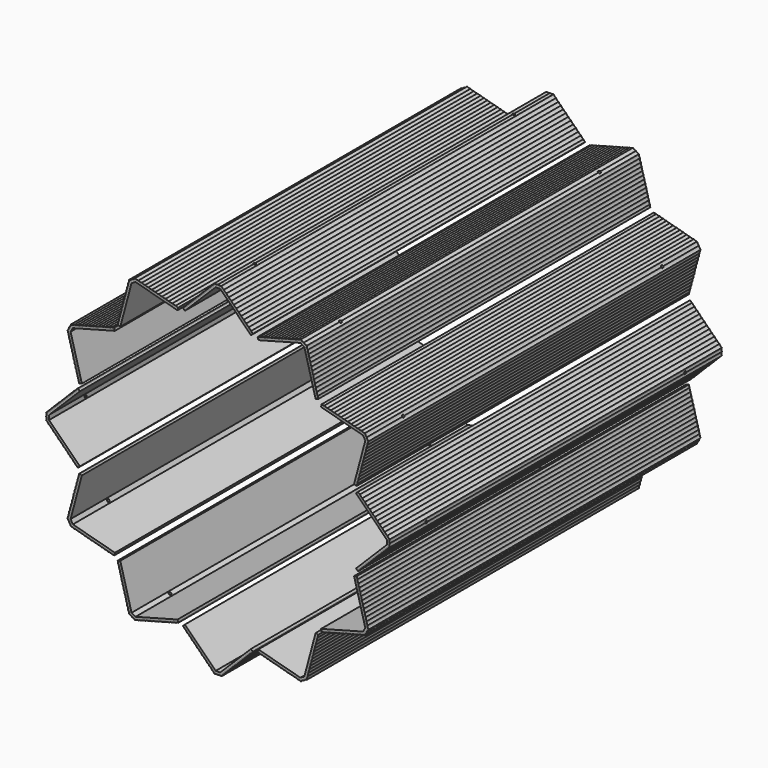
from build123d import *

# Parameters (mm, degrees)
F1_DEPTH = 749.3
F2_DEPTH = 749.3
F3_DEPTH = 749.3
F4_R     = 4.7625
F5_DEPTH = 10.8341
F7_COUNT = 12


with BuildPart() as f1:
    # F0 (on Front) → F1 (new body, symmetric)
    with BuildSketch(Plane.XZ):
        Polygon((8.2127830575, 0), (0, 0), (-8.2127830575, 0), (-119.3411055301, 111.1283224727), (-123.5887666754, 106.8806613274), (-10.701005348, -6.0071), (0, -6.0071), (10.701005348, -6.0071), (123.5887666754, 106.8806613274), (119.3411055301, 111.1283224727), align=None)
        with BuildLine():
            Line((126.3344906062, 104.1349373966), (124.3071871651, 106.1622408377))
            Line((124.3071871651, 106.1622408377), (11.1218463274, -7.0231))
            Line((11.1218463274, -7.0231), (0, -7.0231))
            Line((0, -7.0231), (-11.1218463274, -7.0231))
            Line((-11.1218463274, -7.0231), (-124.3071871651, 106.1622408377))
            Line((-124.3071871651, 106.1622408377), (-126.3344906062, 104.1349373966))
            ThreePointArc((-126.3344906062, 104.1349373966), (-122.9158165988, 100.9260301236), (-120.4630734528, 96.9299734528))
            ThreePointArc((-120.4630734528, 96.9299734528), (-115.136915248, 93.2758755366), (-111.4828173318, 87.9497173318))
            ThreePointArc((-111.4828173318, 87.9497173318), (-106.1566591269, 84.2956194155), (-102.5025612107, 78.9694612107))
            ThreePointArc((-102.5025612107, 78.9694612107), (-97.1764030059, 75.3153632944), (-93.5223050896, 69.9892050896))
            ThreePointArc((-93.5223050896, 69.9892050896), (-88.1961468848, 66.3351071734), (-84.5420489686, 61.0089489686))
            ThreePointArc((-84.5420489686, 61.0089489686), (-79.2158907637, 57.3548510523), (-75.5617928475, 52.0286928475))
            ThreePointArc((-75.5617928475, 52.0286928475), (-70.2356346427, 48.3745949312), (-66.5815367264, 43.0484367264))
            ThreePointArc((-66.5815367264, 43.0484367264), (-61.2553785216, 39.3943388102), (-57.6012806053, 34.0681806053))
            ThreePointArc((-57.6012806053, 34.0681806053), (-52.2751224005, 30.4140826891), (-48.6210244843, 25.0879244843))
            ThreePointArc((-48.6210244843, 25.0879244843), (-43.2948662795, 21.433826568), (-39.6407683632, 16.1076683632))
            ThreePointArc((-39.6407683632, 16.1076683632), (-34.3146101584, 12.453570447), (-30.6605122421, 7.1274122421))
            ThreePointArc((-30.6605122421, 7.1274122421), (-25.3343540373, 3.4733143259), (-21.6802561211, -1.8528438789))
            ThreePointArc((-21.6802561211, -1.8528438789), (-16.3540979162, -5.5069417952), (-12.7, -10.8331))
            ThreePointArc((-12.7, -10.8331), (-6.35, -9.6507748314), (0, -10.8331))
            ThreePointArc((0, -10.8331), (6.35, -9.6507748314), (12.7, -10.8331))
            ThreePointArc((12.7, -10.8331), (16.3540979162, -5.5069417952), (21.6802561211, -1.8528438789))
            ThreePointArc((21.6802561211, -1.8528438789), (25.3343540373, 3.4733143259), (30.6605122421, 7.1274122421))
            ThreePointArc((30.6605122421, 7.1274122421), (34.3146101584, 12.453570447), (39.6407683632, 16.1076683632))
            ThreePointArc((39.6407683632, 16.1076683632), (43.2948662795, 21.433826568), (48.6210244843, 25.0879244843))
            ThreePointArc((48.6210244843, 25.0879244843), (52.2751224005, 30.4140826891), (57.6012806053, 34.0681806053))
            ThreePointArc((57.6012806053, 34.0681806053), (61.2553785216, 39.3943388102), (66.5815367264, 43.0484367264))
            ThreePointArc((66.5815367264, 43.0484367264), (70.2356346427, 48.3745949312), (75.5617928475, 52.0286928475))
            ThreePointArc((75.5617928475, 52.0286928475), (79.2158907637, 57.3548510523), (84.5420489686, 61.0089489686))
            ThreePointArc((84.5420489686, 61.0089489686), (88.1961468848, 66.3351071734), (93.5223050896, 69.9892050896))
            ThreePointArc((93.5223050896, 69.9892050896), (97.1764030059, 75.3153632944), (102.5025612107, 78.9694612107))
            ThreePointArc((102.5025612107, 78.9694612107), (106.1566591269, 84.2956194155), (111.4828173318, 87.9497173318))
            ThreePointArc((111.4828173318, 87.9497173318), (115.136915248, 93.2758755366), (120.4630734528, 96.9299734528))
            ThreePointArc((120.4630734528, 96.9299734528), (122.9158165988, 100.9260301236), (126.3344906062, 104.1349373966))
        make_face()
        Polygon((124.3071871651, 106.1622408377), (123.5887666754, 106.8806613274), (10.701005348, -6.0071), (0, -6.0071), (-10.701005348, -6.0071), (-123.5887666754, 106.8806613274), (-124.3071871651, 106.1622408377), (-11.1218463274, -7.0231), (0, -7.0231), (11.1218463274, -7.0231), align=None)
    extrude(amount=F1_DEPTH, both=True)


with BuildPart() as f2:
    # F0 (on Front) → F2 (new body, symmetric)
    with BuildSketch(Plane.XZ):
        Polygon((124.3071871651, 106.1622408377), (123.5887666754, 106.8806613274), (10.701005348, -6.0071), (0, -6.0071), (-10.701005348, -6.0071), (-123.5887666754, 106.8806613274), (-124.3071871651, 106.1622408377), (-11.1218463274, -7.0231), (0, -7.0231), (11.1218463274, -7.0231), align=None)
    extrude(amount=F2_DEPTH, both=True)


with BuildPart() as f3:
    # F0 (on Front) → F3 (new body, symmetric)
    with BuildSketch(Plane.XZ):
        with BuildLine():
            Line((126.3344906062, 104.1349373966), (124.3071871651, 106.1622408377))
            Line((124.3071871651, 106.1622408377), (11.1218463274, -7.0231))
            Line((11.1218463274, -7.0231), (0, -7.0231))
            Line((0, -7.0231), (-11.1218463274, -7.0231))
            Line((-11.1218463274, -7.0231), (-124.3071871651, 106.1622408377))
            Line((-124.3071871651, 106.1622408377), (-126.3344906062, 104.1349373966))
            ThreePointArc((-126.3344906062, 104.1349373966), (-122.9158165988, 100.9260301236), (-120.4630734528, 96.9299734528))
            ThreePointArc((-120.4630734528, 96.9299734528), (-115.136915248, 93.2758755366), (-111.4828173318, 87.9497173318))
            ThreePointArc((-111.4828173318, 87.9497173318), (-106.1566591269, 84.2956194155), (-102.5025612107, 78.9694612107))
            ThreePointArc((-102.5025612107, 78.9694612107), (-97.1764030059, 75.3153632944), (-93.5223050896, 69.9892050896))
            ThreePointArc((-93.5223050896, 69.9892050896), (-88.1961468848, 66.3351071734), (-84.5420489686, 61.0089489686))
            ThreePointArc((-84.5420489686, 61.0089489686), (-79.2158907637, 57.3548510523), (-75.5617928475, 52.0286928475))
            ThreePointArc((-75.5617928475, 52.0286928475), (-70.2356346427, 48.3745949312), (-66.5815367264, 43.0484367264))
            ThreePointArc((-66.5815367264, 43.0484367264), (-61.2553785216, 39.3943388102), (-57.6012806053, 34.0681806053))
            ThreePointArc((-57.6012806053, 34.0681806053), (-52.2751224005, 30.4140826891), (-48.6210244843, 25.0879244843))
            ThreePointArc((-48.6210244843, 25.0879244843), (-43.2948662795, 21.433826568), (-39.6407683632, 16.1076683632))
            ThreePointArc((-39.6407683632, 16.1076683632), (-34.3146101584, 12.453570447), (-30.6605122421, 7.1274122421))
            ThreePointArc((-30.6605122421, 7.1274122421), (-25.3343540373, 3.4733143259), (-21.6802561211, -1.8528438789))
            ThreePointArc((-21.6802561211, -1.8528438789), (-16.3540979162, -5.5069417952), (-12.7, -10.8331))
            ThreePointArc((-12.7, -10.8331), (-6.35, -9.6507748314), (0, -10.8331))
            ThreePointArc((0, -10.8331), (6.35, -9.6507748314), (12.7, -10.8331))
            ThreePointArc((12.7, -10.8331), (16.3540979162, -5.5069417952), (21.6802561211, -1.8528438789))
            ThreePointArc((21.6802561211, -1.8528438789), (25.3343540373, 3.4733143259), (30.6605122421, 7.1274122421))
            ThreePointArc((30.6605122421, 7.1274122421), (34.3146101584, 12.453570447), (39.6407683632, 16.1076683632))
            ThreePointArc((39.6407683632, 16.1076683632), (43.2948662795, 21.433826568), (48.6210244843, 25.0879244843))
            ThreePointArc((48.6210244843, 25.0879244843), (52.2751224005, 30.4140826891), (57.6012806053, 34.0681806053))
            ThreePointArc((57.6012806053, 34.0681806053), (61.2553785216, 39.3943388102), (66.5815367264, 43.0484367264))
            ThreePointArc((66.5815367264, 43.0484367264), (70.2356346427, 48.3745949312), (75.5617928475, 52.0286928475))
            ThreePointArc((75.5617928475, 52.0286928475), (79.2158907637, 57.3548510523), (84.5420489686, 61.0089489686))
            ThreePointArc((84.5420489686, 61.0089489686), (88.1961468848, 66.3351071734), (93.5223050896, 69.9892050896))
            ThreePointArc((93.5223050896, 69.9892050896), (97.1764030059, 75.3153632944), (102.5025612107, 78.9694612107))
            ThreePointArc((102.5025612107, 78.9694612107), (106.1566591269, 84.2956194155), (111.4828173318, 87.9497173318))
            ThreePointArc((111.4828173318, 87.9497173318), (115.136915248, 93.2758755366), (120.4630734528, 96.9299734528))
            ThreePointArc((120.4630734528, 96.9299734528), (122.9158165988, 100.9260301236), (126.3344906062, 104.1349373966))
        make_face()
    extrude(amount=F3_DEPTH, both=True)


with BuildPart() as f5_tool:
    # F4 (on Top) → F5 (new body, through all)
    with BuildSketch(Plane.XY):
        with Locations((0, 584.2)):
            Circle(F4_R)
        with Locations((0, -584.2)):
            Circle(F4_R)
    extrude(amount=-F5_DEPTH)


with BuildPart() as f1_1:
    add(f1.part)

    # F5: cut by f5_tool
    add(f5_tool.part, mode=Mode.SUBTRACT)


with BuildPart() as f2_1:
    add(f2.part)

    # F5: cut by f5_tool
    add(f5_tool.part, mode=Mode.SUBTRACT)


with BuildPart() as f3_1:
    add(f3.part)

    # F5: cut by f5_tool
    add(f5_tool.part, mode=Mode.SUBTRACT)


with BuildPart() as f7_1:
    # F7: instance of F1
    add(f1_1.part.rotate(Axis((0, 176.1252135038, 609.6), (0, 1, 0)), 1 * 360 / F7_COUNT))


with BuildPart() as f7_2:
    # F7: instance of F1
    add(f1_1.part.rotate(Axis((0, 176.1252135038, 609.6), (0, 1, 0)), 2 * 360 / F7_COUNT))


with BuildPart() as f7_3:
    # F7: instance of F1
    add(f1_1.part.rotate(Axis((0, 176.1252135038, 609.6), (0, 1, 0)), 3 * 360 / F7_COUNT))


with BuildPart() as f7_4:
    # F7: instance of F1
    add(f1_1.part.rotate(Axis((0, 176.1252135038, 609.6), (0, 1, 0)), 4 * 360 / F7_COUNT))


with BuildPart() as f7_5:
    # F7: instance of F1
    add(f1_1.part.rotate(Axis((0, 176.1252135038, 609.6), (0, 1, 0)), 5 * 360 / F7_COUNT))


with BuildPart() as f7_6:
    # F7: instance of F1
    add(f1_1.part.rotate(Axis((0, 176.1252135038, 609.6), (0, 1, 0)), 6 * 360 / F7_COUNT))


with BuildPart() as f7_7:
    # F7: instance of F1
    add(f1_1.part.rotate(Axis((0, 176.1252135038, 609.6), (0, 1, 0)), 7 * 360 / F7_COUNT))


with BuildPart() as f7_8:
    # F7: instance of F1
    add(f1_1.part.rotate(Axis((0, 176.1252135038, 609.6), (0, 1, 0)), 8 * 360 / F7_COUNT))


with BuildPart() as f7_9:
    # F7: instance of F1
    add(f1_1.part.rotate(Axis((0, 176.1252135038, 609.6), (0, 1, 0)), 9 * 360 / F7_COUNT))


with BuildPart() as f7_10:
    # F7: instance of F1
    add(f1_1.part.rotate(Axis((0, 176.1252135038, 609.6), (0, 1, 0)), 10 * 360 / F7_COUNT))


with BuildPart() as f7_11:
    # F7: instance of F1
    add(f1_1.part.rotate(Axis((0, 176.1252135038, 609.6), (0, 1, 0)), 11 * 360 / F7_COUNT))


with BuildPart() as f7_12:
    # F7: instance of F2
    add(f2_1.part.rotate(Axis((0, 176.1252135038, 609.6), (0, 1, 0)), 1 * 360 / F7_COUNT))


with BuildPart() as f7_13:
    # F7: instance of F2
    add(f2_1.part.rotate(Axis((0, 176.1252135038, 609.6), (0, 1, 0)), 2 * 360 / F7_COUNT))


with BuildPart() as f7_14:
    # F7: instance of F2
    add(f2_1.part.rotate(Axis((0, 176.1252135038, 609.6), (0, 1, 0)), 3 * 360 / F7_COUNT))


with BuildPart() as f7_15:
    # F7: instance of F2
    add(f2_1.part.rotate(Axis((0, 176.1252135038, 609.6), (0, 1, 0)), 4 * 360 / F7_COUNT))


with BuildPart() as f7_16:
    # F7: instance of F2
    add(f2_1.part.rotate(Axis((0, 176.1252135038, 609.6), (0, 1, 0)), 5 * 360 / F7_COUNT))


with BuildPart() as f7_17:
    # F7: instance of F2
    add(f2_1.part.rotate(Axis((0, 176.1252135038, 609.6), (0, 1, 0)), 6 * 360 / F7_COUNT))


with BuildPart() as f7_18:
    # F7: instance of F2
    add(f2_1.part.rotate(Axis((0, 176.1252135038, 609.6), (0, 1, 0)), 7 * 360 / F7_COUNT))


with BuildPart() as f7_19:
    # F7: instance of F2
    add(f2_1.part.rotate(Axis((0, 176.1252135038, 609.6), (0, 1, 0)), 8 * 360 / F7_COUNT))


with BuildPart() as f7_20:
    # F7: instance of F2
    add(f2_1.part.rotate(Axis((0, 176.1252135038, 609.6), (0, 1, 0)), 9 * 360 / F7_COUNT))


with BuildPart() as f7_21:
    # F7: instance of F2
    add(f2_1.part.rotate(Axis((0, 176.1252135038, 609.6), (0, 1, 0)), 10 * 360 / F7_COUNT))


with BuildPart() as f7_22:
    # F7: instance of F2
    add(f2_1.part.rotate(Axis((0, 176.1252135038, 609.6), (0, 1, 0)), 11 * 360 / F7_COUNT))


with BuildPart() as f7_23:
    # F7: instance of F3
    add(f3_1.part.rotate(Axis((0, 176.1252135038, 609.6), (0, 1, 0)), 1 * 360 / F7_COUNT))


with BuildPart() as f7_24:
    # F7: instance of F3
    add(f3_1.part.rotate(Axis((0, 176.1252135038, 609.6), (0, 1, 0)), 2 * 360 / F7_COUNT))


with BuildPart() as f7_25:
    # F7: instance of F3
    add(f3_1.part.rotate(Axis((0, 176.1252135038, 609.6), (0, 1, 0)), 3 * 360 / F7_COUNT))


with BuildPart() as f7_26:
    # F7: instance of F3
    add(f3_1.part.rotate(Axis((0, 176.1252135038, 609.6), (0, 1, 0)), 4 * 360 / F7_COUNT))


with BuildPart() as f7_27:
    # F7: instance of F3
    add(f3_1.part.rotate(Axis((0, 176.1252135038, 609.6), (0, 1, 0)), 5 * 360 / F7_COUNT))


with BuildPart() as f7_28:
    # F7: instance of F3
    add(f3_1.part.rotate(Axis((0, 176.1252135038, 609.6), (0, 1, 0)), 6 * 360 / F7_COUNT))


with BuildPart() as f7_29:
    # F7: instance of F3
    add(f3_1.part.rotate(Axis((0, 176.1252135038, 609.6), (0, 1, 0)), 7 * 360 / F7_COUNT))


with BuildPart() as f7_30:
    # F7: instance of F3
    add(f3_1.part.rotate(Axis((0, 176.1252135038, 609.6), (0, 1, 0)), 8 * 360 / F7_COUNT))


with BuildPart() as f7_31:
    # F7: instance of F3
    add(f3_1.part.rotate(Axis((0, 176.1252135038, 609.6), (0, 1, 0)), 9 * 360 / F7_COUNT))


with BuildPart() as f7_32:
    # F7: instance of F3
    add(f3_1.part.rotate(Axis((0, 176.1252135038, 609.6), (0, 1, 0)), 10 * 360 / F7_COUNT))


with BuildPart() as f7_33:
    # F7: instance of F3
    add(f3_1.part.rotate(Axis((0, 176.1252135038, 609.6), (0, 1, 0)), 11 * 360 / F7_COUNT))


solid = Compound([f1_1.part, f2_1.part, f3_1.part, f7_1.part, f7_2.part, f7_3.part, f7_4.part, f7_5.part, f7_6.part, f7_7.part, f7_8.part, f7_9.part, f7_10.part, f7_11.part, f7_12.part, f7_13.part, f7_14.part, f7_15.part, f7_16.part, f7_17.part, f7_18.part, f7_19.part, f7_20.part, f7_21.part, f7_22.part, f7_23.part, f7_24.part, f7_25.part, f7_26.part, f7_27.part, f7_28.part, f7_29.part, f7_30.part, f7_31.part, f7_32.part, f7_33.part])
